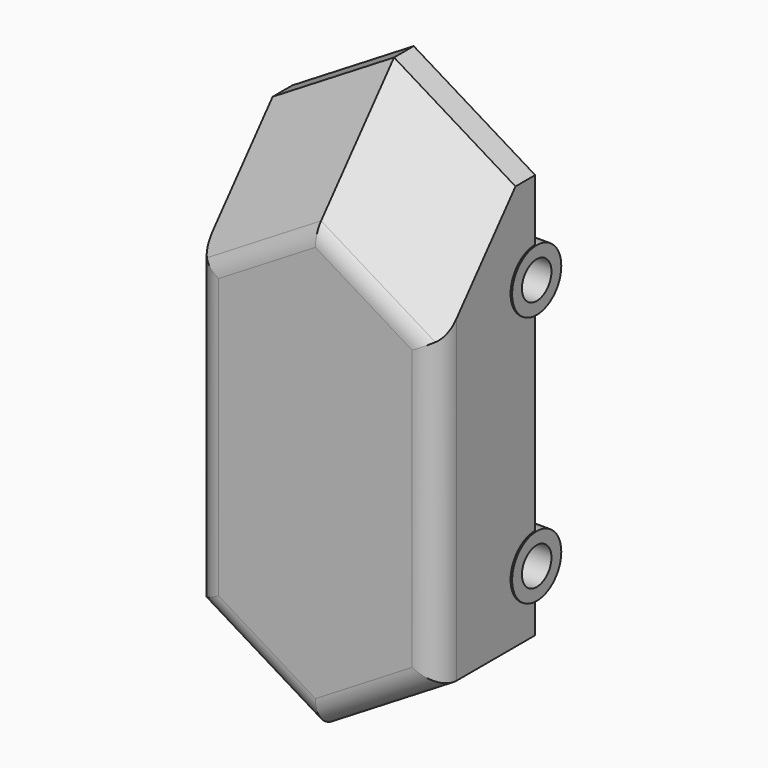
from build123d import *

# Parameters (mm, degrees)
F1_DEPTH       = 25.4
F2_SIZE        = 20.32
F5_R           = 6.35
F6_DEPTH       = 25.4
F6_DEPTH_BACK  = 25.4
F7_R           = 3.81
F8_DEPTH       = 46.228
F8_DEPTH_BACK  = 55.88
F9_R           = 6.35
F10_DEPTH      = 25.4
F10_DEPTH_BACK = 25.4
F11_R          = 3.81
F12_DEPTH      = 41.402
F12_DEPTH_BACK = 45.212
F13_R          = 5.08


# Not quite as in the source:
# - a feature of the source that left no trace in its solid (it failed there, or was rolled back) is left out


with BuildPart() as f1:
    # F0 (on Front) → F1 (new body)
    with BuildSketch(Plane.XZ):
        Polygon((0, 57.15), (-25.0849546432, 41.8481773181), (-25.0849546432, -41.8481773181), (0, -57.15), (25.0849546432, -41.8481773181), (25.0849546432, 41.8481773181), align=None)
    extrude(amount=F1_DEPTH)

    # F2
    f2_edges = [f1.edges().sort_by_distance(p)[0] for p in [
        (-12.542477, -25.4, 49.499089),
        (12.542477, -25.4, 49.499089),
    ]]
    chamfer(f2_edges, length=F2_SIZE)

    # F5 (on Right) → F6 (join, two sides)
    with BuildSketch(Plane.YZ) as f6_sk:
        with Locations((0, -29.1547831148)):
            Circle(F5_R)
    extrude(amount=-F6_DEPTH)
    extrude(f6_sk.sketch, amount=F6_DEPTH_BACK)

    # F7 (on Right) → F8 (cut, two sides)
    with BuildSketch(Plane.YZ) as f8_sk:
        with Locations((0, -29.1547831148)):
            Circle(F7_R)
    extrude(amount=-F8_DEPTH, mode=Mode.SUBTRACT)
    extrude(f8_sk.sketch, amount=F8_DEPTH_BACK, mode=Mode.SUBTRACT)

    # F9 (on Right) → F10 (join, two sides)
    with BuildSketch(Plane.YZ) as f10_sk:
        with Locations((0, 22.8599980474)):
            Circle(F9_R)
    extrude(amount=F10_DEPTH)
    extrude(f10_sk.sketch, amount=-F10_DEPTH_BACK)

    # F11 (on Right) → F12 (cut, two sides)
    with BuildSketch(Plane.YZ) as f12_sk:
        with Locations((0, 22.8599980474)):
            Circle(F11_R)
    extrude(amount=-F12_DEPTH, mode=Mode.SUBTRACT)
    extrude(f12_sk.sketch, amount=F12_DEPTH_BACK, mode=Mode.SUBTRACT)

    # F13
    f13_edges = [f1.edges().sort_by_distance(p)[0] for p in [
        (-25.084955, -25.4, -11.901086),
        (-12.542477, -25.4, 25.696917),
        (-12.542477, -25.4, -49.499089),
        (12.542477, -25.4, 25.696917),
        (12.542477, -25.4, -49.499089),
        (25.084955, -25.4, -11.901086),
    ]]
    fillet(f13_edges, radius=F13_R)


solid = f1.part
